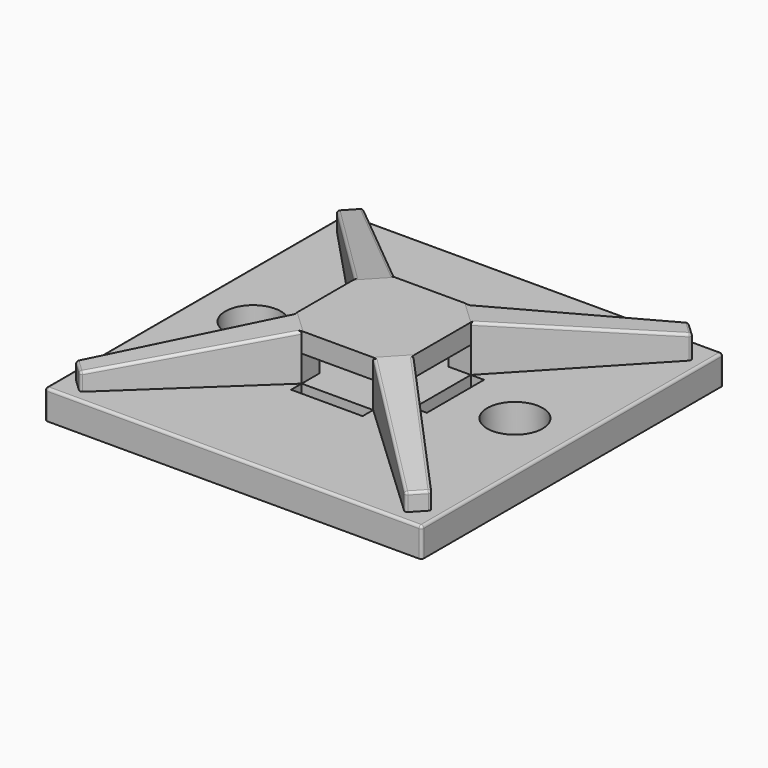
from build123d import *

# Parameters (mm, degrees)
F0_W           = 28.5
F0_H           = 28.5
F1_DEPTH       = 2.2
F3_DEPTH       = 3.5
F3_FACE4_W     = 1.6
F3_FACE4_H     = 3.5
F8_DEPTH       = 21.4958746119
F3_FACE5_W     = 1.6
F3_FACE5_H     = 3.5
F9_DEPTH       = 21.4958746119
F3_FACE6_W     = 1.6
F3_FACE6_H     = 3.5
F10_DEPTH      = 21.4958746119
F3_FACE7_W     = 1.6
F3_FACE7_H     = 3.5
F11_DEPTH      = 21.4958746119
F12_R          = 2.1
F12_W          = 5.4058874503
F12_H          = 1
F13_DEPTH      = 2.201
F14_W          = 5.4058874503
F14_H          = 2
F16_DEPTH      = 18.651
F15_W          = 5.4058874503
F15_H          = 2
F17_DEPTH      = 18.651
F18_T1_DEPTH   = 1.2139704195
F18_T3_DEPTH   = 1.2139704195
F18_T5_DEPTH   = 1.1305618021
F18_T7_DEPTH   = 1.2139704195
F18_T9_DEPTH   = 1.2139704195
F18_T11_DEPTH  = 1.5747546072
F18_T13_DEPTH  = 28.1
F18_T15_DEPTH  = 2.5
F18_T17_DEPTH  = 28.1
F18_T22_DEPTH  = 0.204
F18_T28_DEPTH  = 0.3949972008
F18_T40_DEPTH  = 0.204
F18_T46_DEPTH  = 0.3949972008
F18_T58_DEPTH  = 0.3949972008
F18_T70_DEPTH  = 0.204
F18_T76_DEPTH  = 0.204
F18_T82_DEPTH  = 0.3987751306
F18_S93_W      = 0.204
F18_S93_H      = 0.204
F18_T94_DEPTH  = 0.204
F18_S99_W      = 0.204
F18_S99_H      = 0.204
F18_T100_DEPTH = 0.204
F18_S105_W     = 0.204
F18_S105_H     = 0.204
F18_T106_DEPTH = 0.204
F18_S111_W     = 0.204
F18_S111_H     = 0.204
F18_T112_DEPTH = 0.204
F18_T118_DEPTH = 14.718616179
F18_T123_DEPTH = 13.675330472
F18_T128_DEPTH = 14.718616179
F18_T133_DEPTH = 13.675330472
F18_T138_DEPTH = 13.675330472
F18_T143_DEPTH = 14.718616179
F18_T148_DEPTH = 15.6462597775
F18_T153_DEPTH = 13.6045176404


# Not quite as in the source:
# - a fillet or chamfer that OpenCascade refuses, or shapes differently, is made with other operations: its cross-section is extruded or revolved along the edge and cut away or added
# - a feature names something its author has since deleted; it is built from what else it names


with BuildPart() as f1:
    # F0 (on Top) → F1 (new body)
    with BuildSketch(Plane.XY):
        Rectangle(F0_W, F0_H)
    extrude(amount=F1_DEPTH)

    # F2 (on face) → F3 (join)
    with BuildSketch(Plane.XY.offset(2.2)):
        Polygon((12.3195959493, -13.4509667992), (13.4509667992, -12.3195959493), (4.4, -2.7029437252), (4.4, 2.7029437252), (13.4509667992, 12.3195959493), (12.3195959493, 13.4509667992), (2.7029437252, 4.4), (-2.7029437252, 4.4), (-12.3195959493, 13.4509667992), (-13.4509667992, 12.3195959493), (-4.4, 2.7029437252), (-4.4, -2.7029437252), (-13.4509667992, -12.3195959493), (-12.3195959493, -13.4509667992), (-2.7029437252, -4.4), (2.7029437252, -4.4), align=None)
    extrude(amount=F3_DEPTH)

    # F7 (on face) + F3_face4 (on face) → F8 (cut, through all)
    with BuildSketch(Plane(origin=(0.9842189115, -0.9263236814, 0), x_dir=(0.685364699, 0.7281999927, 0), z_dir=(0.7281999927, -0.685364699, 0))):
        Polygon((4.9838882765, 5.7), (18.1899474919, 3.95), (18.1899474919, 5.7), align=None)
    with BuildSketch(Plane(origin=(12.8852813742, 12.8852813742, 3.95), x_dir=(-0.7071067812, 0.7071067812, 0), z_dir=(0.7071067812, 0.7071067812, 0))):
        Rectangle(F3_FACE4_W, F3_FACE4_H)
    extrude(amount=-F8_DEPTH, dir=(0.7281999927, -0.685364699, 0), mode=Mode.SUBTRACT)

    # F6 (on face) + F3_face5 (on face) → F9 (cut, through all)
    with BuildSketch(Plane(origin=(0.9263236814, 0.9842189115, 0), x_dir=(-0.7281999927, 0.685364699, 0), z_dir=(0.685364699, 0.7281999927, 0))):
        Polygon((4.9838882765, 5.7), (18.1899474919, 3.5), (18.1899474919, 5.7), align=None)
    with BuildSketch(Plane(origin=(-12.8852813742, 12.8852813742, 3.95), x_dir=(-0.7071067812, -0.7071067812, 0), z_dir=(-0.7071067812, 0.7071067812, 0))):
        Rectangle(F3_FACE5_W, F3_FACE5_H)
    extrude(amount=-F9_DEPTH, dir=(0.685364699, 0.7281999927, 0), mode=Mode.SUBTRACT)

    # F5 (on face) + F3_face6 (on face) → F10 (cut, through all)
    with BuildSketch(Plane(origin=(-0.9842189115, 0.9263236814, 0), x_dir=(-0.685364699, -0.7281999927, 0), z_dir=(-0.7281999927, 0.685364699, 0))):
        Polygon((4.9838882765, 5.7), (18.1899474919, 3.5), (18.1899474919, 5.7), align=None)
    with BuildSketch(Plane(origin=(-12.8852813742, -12.8852813742, 3.95), x_dir=(0.7071067812, -0.7071067812, 0), z_dir=(-0.7071067812, -0.7071067812, 0))):
        Rectangle(F3_FACE6_W, F3_FACE6_H)
    extrude(amount=-F10_DEPTH, dir=(-0.7281999927, 0.685364699, 0), mode=Mode.SUBTRACT)

    # F4 (on face) + F3_face7 (on face) → F11 (cut, through all)
    with BuildSketch(Plane(origin=(-0.9263236814, -0.9842189115, 0), x_dir=(0.7281999927, -0.685364699, 0), z_dir=(-0.685364699, -0.7281999927, 0))):
        Polygon((4.9838882765, 5.7), (18.1899474919, 3.5), (18.1899474919, 5.7), align=None)
    with BuildSketch(Plane(origin=(12.8852813742, -12.8852813742, 3.95), x_dir=(0.7071067812, 0.7071067812, 0), z_dir=(0.7071067812, -0.7071067812, 0))):
        Rectangle(F3_FACE7_W, F3_FACE7_H)
    extrude(amount=-F11_DEPTH, dir=(-0.685364699, -0.7281999927, 0), mode=Mode.SUBTRACT)

    # F12 (on face) → F13 (cut, through all)
    with BuildSketch(Plane.XY.offset(2.2)):
        with Locations((-9.9, 0)):
            Circle(F12_R)
        with Locations((9.9, 0)):
            Circle(F12_R)
        with Locations((0, 4.9)):
            Rectangle(F12_W, F12_H)
        with Locations((0, -4.9)):
            Rectangle(F12_W, F12_H)
        Polygon((-4.4, 2.5615270715), (-4.4, 2.7029437252), (-5.4, 2.7029437252), (-5.4, -2.7029437252), (-4.4, -2.7029437252), align=None)
        Polygon((5.4, 2.7029437252), (4.4, 2.7029437252), (4.4, 2.5615270715), (4.4, -2.7029437252), (5.4, -2.7029437252), align=None)
    extrude(amount=-F13_DEPTH, mode=Mode.SUBTRACT)

    # F14 (on face) → F16 (cut, through all)
    with BuildSketch(Plane.XZ.offset(4.4)):
        with Locations((0, 3.2)):
            Rectangle(F14_W, F14_H)
    extrude(amount=-F16_DEPTH, mode=Mode.SUBTRACT)

    # F15 (on face) → F17 (cut, through all)
    with BuildSketch(Plane.YZ.offset(4.4)):
        with Locations((0, 3.2)):
            Rectangle(F15_W, F15_H)
    extrude(amount=-F17_DEPTH, mode=Mode.SUBTRACT)

    # F18: fillet of radius 0.2 on 28 edges, made by hand

    # F18_s2 → F18_t1 (cut)
    with BuildSketch(Plane(origin=(-0.8385789129, 0.7892507416, 0), x_dir=(0, 0, 1), z_dir=(0.7281999927, -0.685364699, 0))):
        with BuildLine():
            ThreePointArc((3.5278430327, 18.0228126109), (3.4598424584, 18.142546679), (3.3305618021, 18.1899474919))
            Line((3.3305618021, 18.1899474919), (3.5, 18.1899474919))
            Line((3.5, 18.1899474919), (3.5278430327, 18.0228126109))
        make_face()
    extrude(amount=F18_T1_DEPTH, mode=Mode.SUBTRACT)

    # F18_s4 → F18_t3 (cut)
    with BuildSketch(Plane(origin=(-0.7892507416, -0.8385789129, 0), x_dir=(0, 0, 1), z_dir=(0.685364699, 0.7281999927, 0))):
        with BuildLine():
            ThreePointArc((3.5278430327, 18.0228126109), (3.4598424584, 18.142546679), (3.3305618021, 18.1899474919))
            Line((3.3305618021, 18.1899474919), (3.5, 18.1899474919))
            Line((3.5, 18.1899474919), (3.5278430327, 18.0228126109))
        make_face()
    extrude(amount=F18_T3_DEPTH, mode=Mode.SUBTRACT)

    # F18_s6 → F18_t5 (cut)
    with BuildSketch(Plane.XY.offset(2.2)):
        with BuildLine():
            ThreePointArc((12.4566688891, -13.3053268006), (12.3170867159, -13.3681620967), (12.1739559508, -13.3138938594))
            Line((12.1739559508, -13.3138938594), (12.3195959493, -13.4509667992))
            Line((12.3195959493, -13.4509667992), (12.4566688891, -13.3053268006))
        make_face()
        with BuildLine():
            ThreePointArc((-13.3053268006, -12.4566688891), (-13.3681620967, -12.3170867159), (-13.3138938594, -12.1739559508))
            Line((-13.3138938594, -12.1739559508), (-13.4509667992, -12.3195959493))
            Line((-13.4509667992, -12.3195959493), (-13.3053268006, -12.4566688891))
        make_face()
        with BuildLine():
            ThreePointArc((-12.4566688891, 13.3053268006), (-12.3170867159, 13.3681620967), (-12.1739559508, 13.3138938594))
            Line((-12.1739559508, 13.3138938594), (-12.3195959493, 13.4509667992))
            Line((-12.3195959493, 13.4509667992), (-12.4566688891, 13.3053268006))
        make_face()
        with BuildLine():
            ThreePointArc((-13.2886813603, 12.1471676704), (-13.3430413617, 12.2842406102), (-13.2886813603, 12.42131355))
            Line((-13.2886813603, 12.42131355), (-13.417691186, 12.2842406102))
            Line((-13.417691186, 12.2842406102), (-13.2886813603, 12.1471676704))
        make_face()
        with BuildLine():
            ThreePointArc((-12.1471676704, -13.2886813603), (-12.2842406102, -13.3430413617), (-12.42131355, -13.2886813603))
            Line((-12.42131355, -13.2886813603), (-12.2842406102, -13.417691186))
            Line((-12.2842406102, -13.417691186), (-12.1471676704, -13.2886813603))
        make_face()
        with BuildLine():
            ThreePointArc((13.2886813603, -12.1471676704), (13.3430413617, -12.2842406102), (13.2886813603, -12.42131355))
            Line((13.2886813603, -12.42131355), (13.417691186, -12.2842406102))
            Line((13.417691186, -12.2842406102), (13.2886813603, -12.1471676704))
        make_face()
    extrude(amount=F18_T5_DEPTH, mode=Mode.SUBTRACT)

    # F18_s8 → F18_t7 (cut)
    with BuildSketch(Plane(origin=(0.7892507416, 0.8385789129, 0), x_dir=(0, 0, 1), z_dir=(-0.685364699, -0.7281999927, 0))):
        with BuildLine():
            ThreePointArc((3.3305618021, 18.1899474919), (3.4598424584, 18.142546679), (3.5278430327, 18.0228126109))
            Line((3.5278430327, 18.0228126109), (3.5, 18.1899474919))
            Line((3.5, 18.1899474919), (3.3305618021, 18.1899474919))
        make_face()
    extrude(amount=F18_T7_DEPTH, mode=Mode.SUBTRACT)

    # F18_s10 → F18_t9 (cut)
    with BuildSketch(Plane(origin=(0.8385789129, -0.7892507416, 0), x_dir=(0, 0, 1), z_dir=(-0.7281999927, 0.685364699, 0))):
        with BuildLine():
            ThreePointArc((3.9730213803, 18.0162207993), (3.9065600292, 18.1403713289), (3.7747546072, 18.1899474919))
            Line((3.7747546072, 18.1899474919), (3.95, 18.1899474919))
            Line((3.95, 18.1899474919), (3.9730213803, 18.0162207993))
        make_face()
    extrude(amount=F18_T9_DEPTH, mode=Mode.SUBTRACT)

    # F18_s12 → F18_t11 (cut)
    with BuildSketch(Plane.XY.offset(2.2)):
        with BuildLine():
            ThreePointArc((13.3053268006, 12.4566688891), (13.3681620967, 12.3170867159), (13.3138938594, 12.1739559508))
            Line((13.3138938594, 12.1739559508), (13.4509667992, 12.3195959493))
            Line((13.4509667992, 12.3195959493), (13.3053268006, 12.4566688891))
        make_face()
        with BuildLine():
            ThreePointArc((12.1471676704, 13.2886813603), (12.2842406102, 13.3430413617), (12.42131355, 13.2886813603))
            Line((12.42131355, 13.2886813603), (12.2842406102, 13.417691186))
            Line((12.2842406102, 13.417691186), (12.1471676704, 13.2886813603))
        make_face()
    extrude(amount=F18_T11_DEPTH, mode=Mode.SUBTRACT)

    # F18_s14 → F18_t13 (cut)
    with BuildSketch(Plane.YZ.offset(-14.05)):
        with BuildLine():
            ThreePointArc((14.25, 2), (14.1914213562, 2.1414213562), (14.05, 2.2))
            Line((14.05, 2.2), (14.25, 2.2))
            Line((14.25, 2.2), (14.25, 2))
        make_face()
        with BuildLine():
            ThreePointArc((-14.25, 2), (-14.1914213562, 2.1414213562), (-14.05, 2.2))
            Line((-14.05, 2.2), (-14.25, 2.2))
            Line((-14.25, 2.2), (-14.25, 2))
        make_face()
    extrude(amount=F18_T13_DEPTH, mode=Mode.SUBTRACT)

    # F18_s16 → F18_t15 (cut)
    with BuildSketch(Plane.XY.offset(-0.5)):
        with BuildLine():
            ThreePointArc((-14.05, 14.25), (-14.1914213562, 14.1914213562), (-14.25, 14.05))
            Line((-14.25, 14.05), (-14.25, 14.25))
            Line((-14.25, 14.25), (-14.05, 14.25))
        make_face()
        with BuildLine():
            ThreePointArc((14.05, 14.25), (14.1914213562, 14.1914213562), (14.25, 14.05))
            Line((14.25, 14.05), (14.25, 14.25))
            Line((14.25, 14.25), (14.05, 14.25))
        make_face()
        with BuildLine():
            ThreePointArc((14.05, -14.25), (14.1914213562, -14.1914213562), (14.25, -14.05))
            Line((14.25, -14.05), (14.25, -14.25))
            Line((14.25, -14.25), (14.05, -14.25))
        make_face()
        with BuildLine():
            ThreePointArc((-14.05, -14.25), (-14.1914213562, -14.1914213562), (-14.25, -14.05))
            Line((-14.25, -14.05), (-14.25, -14.25))
            Line((-14.25, -14.25), (-14.05, -14.25))
        make_face()
    extrude(amount=F18_T15_DEPTH, mode=Mode.SUBTRACT)

    # F18_s18 → F18_t17 (cut)
    with BuildSketch(Plane.XZ.offset(-14.05)):
        with BuildLine():
            ThreePointArc((-14.05, 2.2), (-14.1914213562, 2.1414213562), (-14.25, 2))
            Line((-14.25, 2), (-14.25, 2.2))
            Line((-14.25, 2.2), (-14.05, 2.2))
        make_face()
        with BuildLine():
            ThreePointArc((14.25, 2), (14.1914213562, 2.1414213562), (14.05, 2.2))
            Line((14.05, 2.2), (14.25, 2.2))
            Line((14.25, 2.2), (14.25, 2))
        make_face()
    extrude(amount=F18_T17_DEPTH, mode=Mode.SUBTRACT)


with BuildPart() as f18_tool20:
    # F18_s21 → F18_t22 (new body)
    with BuildSketch(Plane(origin=(-0.8385789129, 0.7892507416, 0), x_dir=(0, 0, 1), z_dir=(-0.7281999927, 0.685364699, 0))):
        Polygon((3.3305618021, -17.9899474919), (3.5317886573, -18.0234699133), (3.503388764, -18.1939474919), (3.3305618021, -18.1939474919), align=None)
    extrude(amount=F18_T22_DEPTH)

    # F18_s23 → F18_t24 (revolve, cut)
    with BuildSketch(Plane(origin=(-13.1682538608, -12.3110288906, 3.3305618021), x_dir=(0.5229304796, 0.5556136346, -0.6464032817), z_dir=(0.4430219906, 0.470710865, 0.7629959354))):
        with BuildLine():
            ThreePointArc((0, -0.2), (0.2, 0), (0, 0.2))
            Line((0, 0.2), (0, -0.2))
        make_face()
    revolve(axis=Axis((-13.1682538608, -12.3110288906, 3.3305618021), (-0.7281999927, 0.685364699, 0)), mode=Mode.SUBTRACT)


with BuildPart() as f1_1:
    add(f1.part)

    # F18_t19: cut F18_tool20
    add(f18_tool20.part, mode=Mode.SUBTRACT)


with BuildPart() as f18_tool26:
    # F18_s27 → F18_t28 (new body)
    with BuildSketch(Plane(origin=(-0.8239186246, -11.5300354089, 7.2162762134), x_dir=(0.9974565804, -0.0712767155, 0), z_dir=(-0.0604622048, -0.8461167667, 0.5295571159))):
        Polygon((-10.9775766457, -4.1364572016), (-11.7604753725, -4.242101596), (-11.6548309781, -5.0250003228), (-10.8719322513, -4.9193559284), align=None)
    extrude(amount=F18_T28_DEPTH)

    split(bisect_by=Plane(origin=(-12.3292874796, -11.604035275, -2.8153937798), x_dir=(0.685364699, -0.7281999927, 0), z_dir=(-0.7183365128, -0.6760814238, -0.1640322)), keep=Keep.TOP)

    split(bisect_by=Plane.XY.offset(3.3305618021), keep=Keep.TOP)

    split(bisect_by=Plane(origin=(0.0454343377, -0.0427617296, 0), x_dir=(0, 0, 1), z_dir=(0.7281999927, -0.685364699, 0)), keep=Keep.TOP)

    split(bisect_by=Plane(origin=(-0.7259107916, -0.7712802161, 6.3578763998), x_dir=(-0.7281999927, 0.685364699, 0), z_dir=(0.1126229619, 0.119661897, -0.9864061531)), keep=Keep.TOP)

    split(bisect_by=Plane(origin=(0.9290651402, -0.9871317115, 0), x_dir=(0, 0, 1), z_dir=(-0.685364699, 0.7281999927, 0)), keep=Keep.TOP)

    split(bisect_by=Plane(origin=(-12.4694893465, -13.2488324307, 0), x_dir=(0, 0, 1), z_dir=(0.685364699, 0.7281999927, 0)), keep=Keep.TOP)

    # F18_s35 → F18_t36 (revolve, cut)
    with BuildSketch(Plane(origin=(-12.2842406102, -13.1430413617, 3.3305618021), x_dir=(0.0604622048, 0.8461167667, -0.5295571159), z_dir=(-0.0959818345, 0.5329975771, 0.8406551435))):
        with BuildLine():
            ThreePointArc((0, -0.2), (0.2, 0), (0, 0.2))
            Line((0, 0.2), (0, -0.2))
        make_face()
    revolve(axis=Axis((-12.2842406102, -13.1430413617, 3.3305618021), (-0.9935450716, 0, -0.1134380482)), mode=Mode.SUBTRACT)


with BuildPart() as f1_2:
    add(f1_1.part)

    # F18_t25: cut F18_tool26
    add(f18_tool26.part, mode=Mode.SUBTRACT)


with BuildPart() as f18_tool38:
    # F18_s39 → F18_t40 (new body)
    with BuildSketch(Plane(origin=(-0.7892507416, -0.8385789129, 0), x_dir=(0, 0, 1), z_dir=(-0.685364699, -0.7281999927, 0))):
        Polygon((3.3305618021, -17.9899474919), (3.5317886573, -18.0234699133), (3.503388764, -18.1939474919), (3.3305618021, -18.1939474919), align=None)
    extrude(amount=F18_T40_DEPTH)

    # F18_s41 → F18_t42 (revolve, cut)
    with BuildSketch(Plane(origin=(12.3110288906, -13.1682538608, 3.3305618021), x_dir=(-0.5556136346, 0.5229304796, -0.6464032817), z_dir=(-0.470710865, 0.4430219906, 0.7629959354))):
        with BuildLine():
            ThreePointArc((0, -0.2), (0.2, 0), (0, 0.2))
            Line((0, 0.2), (0, -0.2))
        make_face()
    revolve(axis=Axis((12.3110288906, -13.1682538608, 3.3305618021), (-0.685364699, -0.7281999927, 0)), mode=Mode.SUBTRACT)


with BuildPart() as f1_3:
    add(f1_2.part)

    # F18_t37: cut F18_tool38
    add(f18_tool38.part, mode=Mode.SUBTRACT)


with BuildPart() as f18_tool44:
    # F18_s45 → F18_t46 (new body)
    with BuildSketch(Plane(origin=(11.5300354089, -0.8239186246, 7.2162762134), x_dir=(0.0712767155, 0.9974565804, 0), z_dir=(0.8461167667, -0.0604622048, 0.5295571159))):
        Polygon((-11.86264205, -4.4647510526), (-11.4321815215, -5.1271670004), (-10.7697655737, -4.6967064718), (-11.2002261023, -4.0342905241), align=None)
    extrude(amount=F18_T46_DEPTH)

    split(bisect_by=Plane(origin=(0.0427617296, 0.0454343377, 0), x_dir=(0, 0, 1), z_dir=(0.685364699, 0.7281999927, 0)), keep=Keep.TOP)

    split(bisect_by=Plane(origin=(11.604035275, -12.3292874796, -2.8153937798), x_dir=(0.7281999927, 0.685364699, 0), z_dir=(0.6760814238, -0.7183365128, -0.1640322)), keep=Keep.TOP)

    split(bisect_by=Plane.XY.offset(3.3305618021), keep=Keep.TOP)

    split(bisect_by=Plane(origin=(13.2488324307, -12.4694893465, 0), x_dir=(0, 0, 1), z_dir=(-0.7281999927, 0.685364699, 0)), keep=Keep.TOP)

    split(bisect_by=Plane(origin=(0.7712802161, -0.7259107916, 6.3578763998), x_dir=(-0.685364699, -0.7281999927, 0), z_dir=(-0.119661897, 0.1126229619, -0.9864061531)), keep=Keep.TOP)

    split(bisect_by=Plane(origin=(0.9871317115, 0.9290651402, 0), x_dir=(0, 0, 1), z_dir=(-0.7281999927, -0.685364699, 0)), keep=Keep.TOP)

    # F18_s53 → F18_t54 (revolve, cut)
    with BuildSketch(Plane(origin=(13.1430413617, -12.2842406102, 3.3305618021), x_dir=(-0.8461167667, 0.0604622048, -0.5295571159), z_dir=(0.2280507575, -0.8569414124, -0.4622166891))):
        with BuildLine():
            ThreePointArc((0, -0.2), (0.2, 0), (0, 0.2))
            Line((0, 0.2), (0, -0.2))
        make_face()
    revolve(axis=Axis((13.1430413617, -12.2842406102, 3.3305618021), (0.481746063, 0.5118551919, -0.7112840455)), mode=Mode.SUBTRACT)


with BuildPart() as f1_4:
    add(f1_3.part)

    # F18_t43: cut F18_tool44
    add(f18_tool44.part, mode=Mode.SUBTRACT)


with BuildPart() as f18_tool56:
    # F18_s57 → F18_t58 (new body)
    with BuildSketch(Plane(origin=(-11.5300354089, 0.8239186246, 7.2162762134), x_dir=(-0.0712767155, -0.9974565804, 0), z_dir=(-0.8461167667, 0.0604622048, 0.5295571159))):
        Polygon((-11.1343577242, -5.1089120425), (-10.7880205316, -4.3988826745), (-11.4980498996, -4.0525454819), (-11.8443870922, -4.7625748499), align=None)
    extrude(amount=F18_T58_DEPTH)

    split(bisect_by=Plane.XY.offset(3.3305618021), keep=Keep.TOP)

    split(bisect_by=Plane(origin=(-0.0427617296, -0.0454343377, 0), x_dir=(0, 0, 1), z_dir=(-0.685364699, -0.7281999927, 0)), keep=Keep.TOP)

    split(bisect_by=Plane(origin=(-11.604035275, 12.3292874796, -2.8153937798), x_dir=(-0.7281999927, -0.685364699, 0), z_dir=(-0.6760814238, 0.7183365128, -0.1640322)), keep=Keep.TOP)

    split(bisect_by=Plane(origin=(-0.9871317115, -0.9290651402, 0), x_dir=(0, 0, 1), z_dir=(0.7281999927, 0.685364699, 0)), keep=Keep.TOP)

    split(bisect_by=Plane(origin=(-13.2488324307, 12.4694893465, 0), x_dir=(0, 0, 1), z_dir=(0.7281999927, -0.685364699, 0)), keep=Keep.TOP)

    split(bisect_by=Plane(origin=(-0.7712802161, 0.7259107916, 6.3578763998), x_dir=(0.685364699, 0.7281999927, 0), z_dir=(0.119661897, -0.1126229619, -0.9864061531)), keep=Keep.TOP)

    # F18_s65 → F18_t66 (revolve, cut)
    with BuildSketch(Plane(origin=(-13.1430413617, 12.2842406102, 3.3305618021), x_dir=(0.8461167667, -0.0604622048, -0.5295571159), z_dir=(-0.2956317272, -0.8799441299, -0.3718873622))):
        with BuildLine():
            ThreePointArc((0, -0.2), (0.2, 0), (0, 0.2))
            Line((0, 0.2), (0, -0.2))
        make_face()
    revolve(axis=Axis((-13.1430413617, 12.2842406102, 3.3305618021), (0.4434955457, -0.4712140173, 0.7624100281)), mode=Mode.SUBTRACT)


with BuildPart() as f1_5:
    add(f1_4.part)

    # F18_t55: cut F18_tool56
    add(f18_tool56.part, mode=Mode.SUBTRACT)


with BuildPart() as f18_tool68:
    # F18_s69 → F18_t70 (new body)
    with BuildSketch(Plane(origin=(0.7892507416, 0.8385789129, 0), x_dir=(0, 0, 1), z_dir=(0.685364699, 0.7281999927, 0))):
        Polygon((3.3305618021, -17.9899474919), (3.5317886573, -18.0234699133), (3.503388764, -18.1939474919), (3.3305618021, -18.1939474919), align=None)
    extrude(amount=F18_T70_DEPTH)

    # F18_s71 → F18_t72 (revolve, cut)
    with BuildSketch(Plane(origin=(-12.3110288906, 13.1682538608, 3.3305618021), x_dir=(0.5556136346, -0.5229304796, -0.6464032817), z_dir=(0.470710865, -0.4430219906, 0.7629959354))):
        with BuildLine():
            ThreePointArc((0, -0.2), (0.2, 0), (0, 0.2))
            Line((0, 0.2), (0, -0.2))
        make_face()
    revolve(axis=Axis((-12.3110288906, 13.1682538608, 3.3305618021), (0.685364699, 0.7281999927, 0)), mode=Mode.SUBTRACT)


with BuildPart() as f1_6:
    add(f1_5.part)

    # F18_t67: cut F18_tool68
    add(f18_tool68.part, mode=Mode.SUBTRACT)


with BuildPart() as f18_tool74:
    # F18_s75 → F18_t76 (new body)
    with BuildSketch(Plane(origin=(0.8385789129, -0.7892507416, 0), x_dir=(0, 0, 1), z_dir=(0.7281999927, -0.685364699, 0))):
        Polygon((3.7747546072, -17.9899474919), (3.9769867158, -18.0167462654), (3.9535049079, -18.1939474919), (3.7747546072, -18.1939474919), align=None)
    extrude(amount=F18_T76_DEPTH)

    # F18_s77 → F18_t78 (revolve, cut)
    with BuildSketch(Plane(origin=(13.1682538608, 12.3110288906, 3.7747546072), x_dir=(-0.5154759388, -0.547693185, -0.6590271099), z_dir=(-0.4516739168, -0.4799035366, 0.752119185))):
        with BuildLine():
            ThreePointArc((0, -0.2), (0.2, 0), (0, 0.2))
            Line((0, 0.2), (0, -0.2))
        make_face()
    revolve(axis=Axis((13.1682538608, 12.3110288906, 3.7747546072), (0.7281999927, -0.685364699, 0)), mode=Mode.SUBTRACT)


with BuildPart() as f1_7:
    add(f1_6.part)

    # F18_t73: cut F18_tool74
    add(f18_tool74.part, mode=Mode.SUBTRACT)


with BuildPart() as f18_tool80:
    # F18_s81 → F18_t82 (new body)
    with BuildSketch(Plane(origin=(0.6686018121, 11.5257681712, 7.3617490574), x_dir=(-0.9983216947, 0.0579119486, 0), z_dir=(0.0488296334, 0.8417551742, 0.5376466252))):
        Polygon((-11.3278650408, -4.7904136354), (-10.9662467989, -4.0795559378), (-11.6771044965, -3.7179376959), (-12.0387227383, -4.4287953935), align=None)
    extrude(amount=F18_T82_DEPTH)

    split(bisect_by=Plane.XY.offset(3.7747546072), keep=Keep.TOP)

    split(bisect_by=Plane(origin=(-0.0454343377, 0.0427617296, 0), x_dir=(0, 0, 1), z_dir=(-0.7281999927, 0.685364699, 0)), keep=Keep.TOP)

    split(bisect_by=Plane(origin=(12.4913591871, 11.7565733526, -2.2689568261), x_dir=(-0.685364699, 0.7281999927, 0), z_dir=(0.721912152, 0.6794467313, -0.1311296458)), keep=Keep.TOP)

    split(bisect_by=Plane(origin=(-0.9290651402, 0.9871317115, 0), x_dir=(0, 0, 1), z_dir=(0.685364699, -0.7281999927, 0)), keep=Keep.TOP)

    split(bisect_by=Plane(origin=(12.4694893465, 13.2488324307, 0), x_dir=(0, 0, 1), z_dir=(-0.685364699, -0.7281999927, 0)), keep=Keep.TOP)

    split(bisect_by=Plane(origin=(0.5680531607, 0.6035564832, 6.2546417684), x_dir=(0.7281999927, -0.685364699, 0), z_dir=(-0.090033987, -0.0956611112, -0.9913338656)), keep=Keep.TOP)

    # F18_s89 → F18_t90 (revolve, cut)
    with BuildSketch(Plane(origin=(12.2842406102, 13.1430413617, 3.7747546072), x_dir=(-0.0488296334, -0.8417551742, -0.5376466252), z_dir=(-0.8756880796, 0.29498289, -0.3823028666))):
        with BuildLine():
            ThreePointArc((0, -0.2), (0.2, 0), (0, 0.2))
            Line((0, 0.2), (0, -0.2))
        make_face()
    revolve(axis=Axis((12.2842406102, 13.1430413617, 3.7747546072), (-0.4804019714, -0.4521430319, 0.7515188784)), mode=Mode.SUBTRACT)


with BuildPart() as f1_8:
    add(f1_7.part)

    # F18_t79: cut F18_tool80
    add(f18_tool80.part, mode=Mode.SUBTRACT)


with BuildPart() as f18_tool92:
    # F18_s93 → F18_t94 (new body)
    with BuildSketch(Plane.XZ.offset(-14.05)):
        with Locations((14.152, 2.102)):
            Rectangle(F18_S93_W, F18_S93_H)
    extrude(amount=-F18_T94_DEPTH)

    # F18_s95 → F18_t96 (revolve, cut)
    with BuildSketch(Plane(origin=(14.05, 14.05, 2), x_dir=(-0.7071067812, 0, -0.7071067812), z_dir=(0.7071067812, 0, -0.7071067812))):
        with BuildLine():
            ThreePointArc((0, -0.2), (0.2, 0), (0, 0.2))
            Line((0, 0.2), (0, -0.2))
        make_face()
    revolve(axis=Axis((14.05, 14.05, 2), (0, 1, 0)), mode=Mode.SUBTRACT)


with BuildPart() as f1_9:
    add(f1_8.part)

    # F18_t91: cut F18_tool92
    add(f18_tool92.part, mode=Mode.SUBTRACT)


with BuildPart() as f18_tool98:
    # F18_s99 → F18_t100 (new body)
    with BuildSketch(Plane.XZ.offset(-14.05)):
        with Locations((-14.152, 2.102)):
            Rectangle(F18_S99_W, F18_S99_H)
    extrude(amount=-F18_T100_DEPTH)

    # F18_s101 → F18_t102 (revolve, cut)
    with BuildSketch(Plane(origin=(-14.05, 14.05, 2), x_dir=(0.7071067812, 0, -0.7071067812), z_dir=(0.7071067812, 0, 0.7071067812))):
        with BuildLine():
            ThreePointArc((0, -0.2), (0.2, 0), (0, 0.2))
            Line((0, 0.2), (0, -0.2))
        make_face()
    revolve(axis=Axis((-14.05, 14.05, 2), (0, 1, 0)), mode=Mode.SUBTRACT)


with BuildPart() as f1_10:
    add(f1_9.part)

    # F18_t97: cut F18_tool98
    add(f18_tool98.part, mode=Mode.SUBTRACT)


with BuildPart() as f18_tool104:
    # F18_s105 → F18_t106 (new body)
    with BuildSketch(Plane.XZ.offset(14.05)):
        with Locations((-14.152, 2.102)):
            Rectangle(F18_S105_W, F18_S105_H)
    extrude(amount=F18_T106_DEPTH)

    # F18_s107 → F18_t108 (revolve, cut)
    with BuildSketch(Plane(origin=(-14.05, -14.05, 2), x_dir=(0.7071067812, 0, -0.7071067812), z_dir=(-0.7071067812, 0, -0.7071067812))):
        with BuildLine():
            ThreePointArc((0, -0.2), (0.2, 0), (0, 0.2))
            Line((0, 0.2), (0, -0.2))
        make_face()
    revolve(axis=Axis((-14.05, -14.05, 2), (0, -1, 0)), mode=Mode.SUBTRACT)


with BuildPart() as f1_11:
    add(f1_10.part)

    # F18_t103: cut F18_tool104
    add(f18_tool104.part, mode=Mode.SUBTRACT)


with BuildPart() as f18_tool110:
    # F18_s111 → F18_t112 (new body)
    with BuildSketch(Plane.XZ.offset(14.05)):
        with Locations((14.152, 2.102)):
            Rectangle(F18_S111_W, F18_S111_H)
    extrude(amount=F18_T112_DEPTH)

    # F18_s113 → F18_t114 (revolve, cut)
    with BuildSketch(Plane(origin=(14.05, -14.05, 2), x_dir=(-0.7071067812, 0, -0.7071067812), z_dir=(-0.7071067812, 0, 0.7071067812))):
        with BuildLine():
            ThreePointArc((0, -0.2), (0.2, 0), (0, 0.2))
            Line((0, 0.2), (0, -0.2))
        make_face()
    revolve(axis=Axis((14.05, -14.05, 2), (0, -1, 0)), mode=Mode.SUBTRACT)


with BuildPart() as f1_12:
    add(f1_11.part)

    # F18_t109: cut F18_tool110
    add(f18_tool110.part, mode=Mode.SUBTRACT)


with BuildPart() as f18_tool116:
    # F18_s117 → F18_t118 (new body)
    with BuildSketch(Plane(origin=(-1.6762488544, -1.7810144078, -0.4074423828), x_dir=(0.7281999927, -0.685364699, 0), z_dir=(-0.6760479562, -0.7183009535, -0.1643255949))):
        with BuildLine():
            ThreePointArc((-1.1515777552, 6.4414954786), (-1.2929991115, 6.3829168348), (-1.3515777552, 6.2414954786))
            Line((-1.3515777552, 6.2414954786), (-1.3515777552, 6.4414954786))
            Line((-1.3515777552, 6.4414954786), (-1.1515777552, 6.4414954786))
        make_face()
    extrude(amount=F18_T118_DEPTH)

    split(bisect_by=Plane.YZ.offset(-4.4), keep=Keep.BOTTOM)


with BuildPart() as f1_13:
    add(f1_12.part)

    # F18_t115: cut F18_tool116
    add(f18_tool116.part, mode=Mode.SUBTRACT)


with BuildPart() as f18_tool121:
    # F18_s122 → F18_t123 (new body)
    with BuildSketch(Plane(origin=(-2.5057982764, -2.3583983778, -0.5721992364), x_dir=(0.685364699, -0.7281999927, 0), z_dir=(-0.7183365128, -0.6760814238, -0.1640322))):
        with BuildLine():
            ThreePointArc((1.1535677533, 6.4303358077), (1.2937009405, 6.371061735), (1.3515777552, 6.2303457082))
            Line((1.3515777552, 6.2303457082), (1.3515777552, 6.4283655126))
            Line((1.3515777552, 6.4283655126), (1.1535677533, 6.4303358077))
        make_face()
    extrude(amount=F18_T123_DEPTH)

    split(bisect_by=Plane.XZ.offset(4.4), keep=Keep.TOP)


with BuildPart() as f1_14:
    add(f1_13.part)

    # F18_t120: cut F18_tool121
    add(f18_tool121.part, mode=Mode.SUBTRACT)


with BuildPart() as f18_tool126:
    # F18_s127 → F18_t128 (new body)
    with BuildSketch(Plane(origin=(1.7810144078, -1.6762488544, -0.4074423828), x_dir=(0.685364699, 0.7281999927, 0), z_dir=(0.7183009535, -0.6760479562, -0.1643255949))):
        with BuildLine():
            ThreePointArc((-1.1515777552, 6.4414954786), (-1.2929991115, 6.3829168348), (-1.3515777552, 6.2414954786))
            Line((-1.3515777552, 6.2414954786), (-1.3515777552, 6.4414954786))
            Line((-1.3515777552, 6.4414954786), (-1.1515777552, 6.4414954786))
        make_face()
    extrude(amount=F18_T128_DEPTH)

    split(bisect_by=Plane.XZ.offset(4.4), keep=Keep.TOP)


with BuildPart() as f1_15:
    add(f1_14.part)

    # F18_t125: cut F18_tool126
    add(f18_tool126.part, mode=Mode.SUBTRACT)


with BuildPart() as f18_tool131:
    # F18_s132 → F18_t133 (new body)
    with BuildSketch(Plane(origin=(2.3583983778, -2.5057982764, -0.5721992364), x_dir=(0.7281999927, 0.685364699, 0), z_dir=(0.6760814238, -0.7183365128, -0.1640322))):
        with BuildLine():
            ThreePointArc((1.1535677533, 6.4303358077), (1.2937009405, 6.371061735), (1.3515777552, 6.2303457082))
            Line((1.3515777552, 6.2303457082), (1.3515777552, 6.4283655126))
            Line((1.3515777552, 6.4283655126), (1.1535677533, 6.4303358077))
        make_face()
    extrude(amount=F18_T133_DEPTH)

    split(bisect_by=Plane.YZ.offset(4.4), keep=Keep.TOP)


with BuildPart() as f1_16:
    add(f1_15.part)

    # F18_t130: cut F18_tool131
    add(f18_tool131.part, mode=Mode.SUBTRACT)


with BuildPart() as f18_tool136:
    # F18_s137 → F18_t138 (new body)
    with BuildSketch(Plane(origin=(-2.3583983778, 2.5057982764, -0.5721992364), x_dir=(-0.7281999927, -0.685364699, 0), z_dir=(-0.6760814238, 0.7183365128, -0.1640322))):
        with BuildLine():
            ThreePointArc((1.3515777552, 6.2303457082), (1.2937009405, 6.371061735), (1.1535677533, 6.4303358077))
            Line((1.1535677533, 6.4303358077), (1.3515777552, 6.4283655126))
            Line((1.3515777552, 6.4283655126), (1.3515777552, 6.2303457082))
        make_face()
    extrude(amount=F18_T138_DEPTH)

    split(bisect_by=Plane.YZ.offset(-4.4), keep=Keep.BOTTOM)


with BuildPart() as f1_17:
    add(f1_16.part)

    # F18_t135: cut F18_tool136
    add(f18_tool136.part, mode=Mode.SUBTRACT)


with BuildPart() as f18_tool141:
    # F18_s142 → F18_t143 (new body)
    with BuildSketch(Plane(origin=(-1.7810144078, 1.6762488544, -0.4074423828), x_dir=(-0.685364699, -0.7281999927, 0), z_dir=(-0.7183009535, 0.6760479562, -0.1643255949))):
        with BuildLine():
            ThreePointArc((-1.3515777552, 6.2414954786), (-1.2929991115, 6.3829168348), (-1.1515777552, 6.4414954786))
            Line((-1.1515777552, 6.4414954786), (-1.3515777552, 6.4414954786))
            Line((-1.3515777552, 6.4414954786), (-1.3515777552, 6.2414954786))
        make_face()
    extrude(amount=F18_T143_DEPTH)

    split(bisect_by=Plane.XZ.offset(-4.4), keep=Keep.BOTTOM)


with BuildPart() as f1_18:
    add(f1_17.part)

    # F18_t140: cut F18_tool141
    add(f18_tool141.part, mode=Mode.SUBTRACT)


with BuildPart() as f18_tool146:
    # F18_s147 → F18_t148 (new body)
    with BuildSketch(Plane(origin=(1.1495249728, 1.2213702836, -0.2222600908), x_dir=(-0.7281999927, 0.685364699, 0), z_dir=(0.6794252364, 0.7218893137, -0.1313665369))):
        with BuildLine():
            ThreePointArc((-1.1515777552, 6.3053191766), (-1.2929991115, 6.2467405329), (-1.3515777552, 6.1053191766))
            Line((-1.3515777552, 6.1053191766), (-1.3515777552, 6.3053191766))
            Line((-1.3515777552, 6.3053191766), (-1.1515777552, 6.3053191766))
        make_face()
    extrude(amount=F18_T148_DEPTH)

    split(bisect_by=Plane.YZ.offset(4.4), keep=Keep.TOP)


with BuildPart() as f1_19:
    add(f1_18.part)

    # F18_t145: cut F18_tool146
    add(f18_tool146.part, mode=Mode.SUBTRACT)


with BuildPart() as f18_tool151:
    # F18_s152 → F18_t153 (new body)
    with BuildSketch(Plane(origin=(2.6700925798, 2.5130283104, -0.4850012472), x_dir=(-0.685364699, 0.7281999927, 0), z_dir=(0.721912152, 0.6794467313, -0.1311296458))):
        with BuildLine():
            ThreePointArc((1.153168616, 6.2963457139), (1.2935604516, 6.2372098201), (1.3515777552, 6.0963520411))
            Line((1.3515777552, 6.0963520411), (1.3515777552, 6.2947674573))
            Line((1.3515777552, 6.2947674573), (1.153168616, 6.2963457139))
        make_face()
    extrude(amount=F18_T153_DEPTH)

    split(bisect_by=Plane.XZ.offset(-4.4), keep=Keep.BOTTOM)


with BuildPart() as f1_20:
    add(f1_19.part)

    # F18_t150: cut F18_tool151
    add(f18_tool151.part, mode=Mode.SUBTRACT)


solid = f1_20.part
